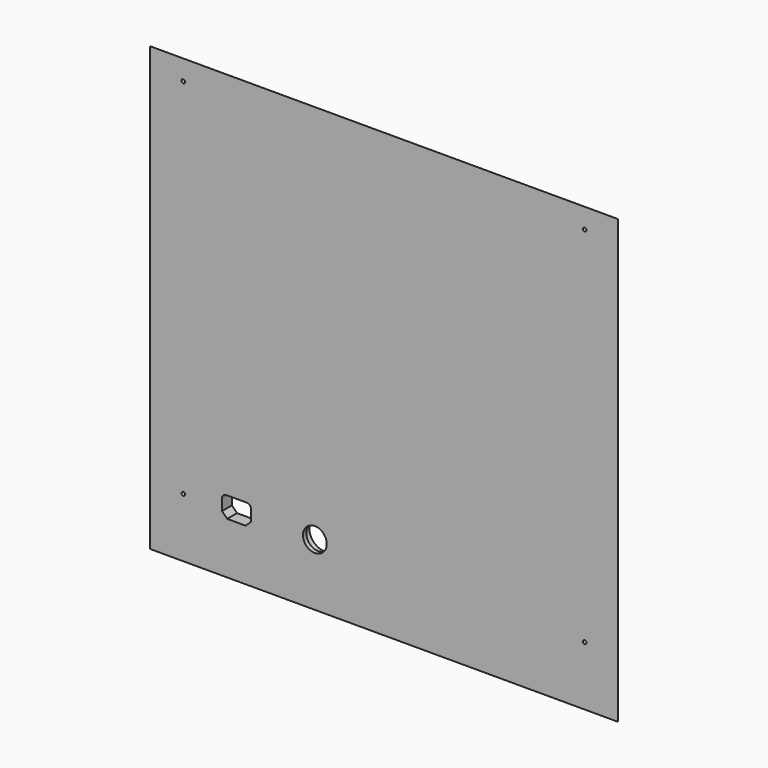
from build123d import *

# Parameters (mm, degrees)
F0_W      = 454
F0_H      = 429
F1_DEPTH  = 12
F2_SIZE   = 11.99999
F3_W      = 28
F3_H      = 20
F3_R      = 11.5
F4_DEPTH  = 25
F5_R      = 4
F6_SIZE   = 5
F8_D      = 3.5
F9_R      = 15
F9_R_2    = 11.5
F10_DEPTH = 8


# Not quite as in the source:
# - a fillet or chamfer is up to 0.001 mm smaller than in the source, because OpenCascade refuses the exact size


with BuildPart() as f1:
    # F0 (on Front) → F1 (new body)
    with BuildSketch(Plane.XZ):
        Rectangle(F0_W, F0_H)
    extrude(amount=F1_DEPTH)

    # F2 (size 12 in the source; OpenCascade refuses exactly that, so slightly less here)
    f2_edges = [f1.edges().sort_by_distance(p)[0] for p in [
        (227, 0, 0),
        (-227, 0, 0),
        (0, 0, 214.5),
    ]]
    chamfer(f2_edges, length=F2_SIZE)

    # F3 (on face) → F4 (cut)
    with BuildSketch(Plane.XZ.offset(12)):
        with Locations((-143, -154.5)):
            Rectangle(F3_W, F3_H)
        with Locations((-67, -154.5)):
            Circle(F3_R)
    extrude(amount=-F4_DEPTH, mode=Mode.SUBTRACT)

    # F5
    f5_edges = [f1.edges().sort_by_distance(p)[0] for p in [
        (-129, -6, -144.5),
        (-157, -6, -144.5),
    ]]
    fillet(f5_edges, radius=F5_R)

    # F6
    f6_edges = [f1.edges().sort_by_distance(p)[0] for p in [
        (-157, -6, -164.5),
        (-129, -6, -164.5),
    ]]
    chamfer(f6_edges, length=F6_SIZE)

    # F8 (through all)
    with Locations(Plane.XZ.offset(12)):
        with Locations((-194.5, 195), (194.5, 195), (194.5, -157), (-194.5, -157)):
            Hole(F8_D / 2)

    # F9 (on face) → F10 (cut)
    with BuildSketch(Plane(origin=(0, 0, 0), x_dir=(-1, 0, 0), z_dir=(0, 1, 0))):
        with Locations((67, -154.5)):
            Circle(F9_R)
        with Locations((67, -154.5)):
            Circle(F9_R_2, mode=Mode.SUBTRACT)
        with Locations((67, -154.5)):
            Circle(F9_R_2)
    extrude(amount=-F10_DEPTH, mode=Mode.SUBTRACT)


solid = f1.part
